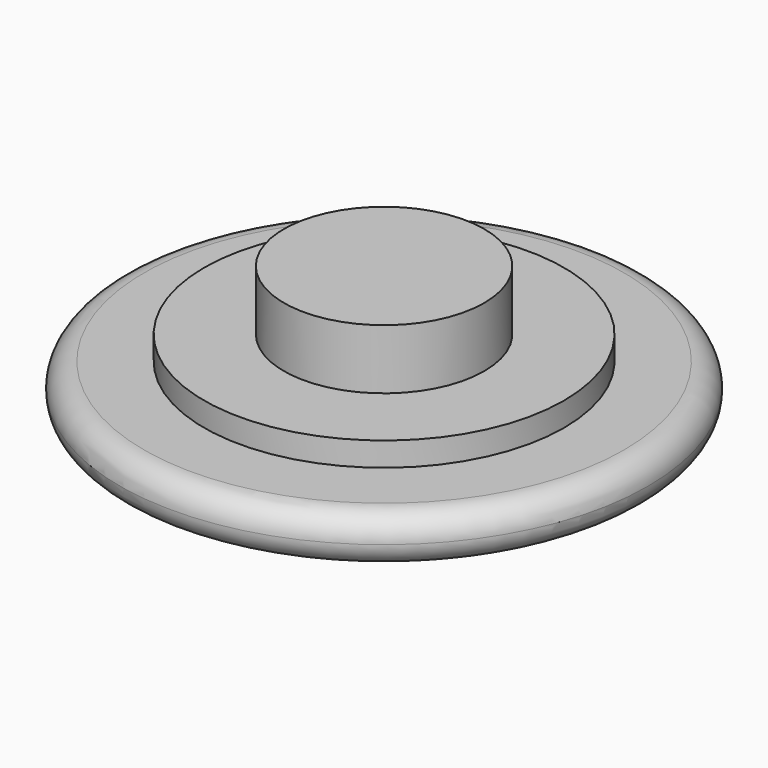
from build123d import *

# Parameters (mm, degrees)
F0_R         = 11
F0_R_2       = 7.5
F1_DEPTH     = 2
F0_R_3       = 4.175
F2_DEPTH     = 3
F3_DEPTH     = 5.5
F4_R         = 0.99999
F5_TEXT_SIZE = 6.3923610263
F6_DEPTH     = 1


# Not quite as in the source:
# - a fillet or chamfer is up to 0.001 mm smaller than in the source, because OpenCascade refuses the exact size
# - Text() gives the source's letters only with a copy of the font that has no kerning and outlines rounded to 1/6400 em; it was checked with that copy


with BuildPart() as f1:
    # F0 (on Top) → F1 (new body)
    with BuildSketch(Plane.XY):
        Circle(F0_R)
        Circle(F0_R_2, mode=Mode.SUBTRACT)
    extrude(amount=F1_DEPTH)

    # F0 (on Top) → F2 (join)
    with BuildSketch(Plane.XY):
        Circle(F0_R_2)
        Circle(F0_R_3, mode=Mode.SUBTRACT)
    extrude(amount=F2_DEPTH)

    # F0 (on Top) → F3 (join)
    with BuildSketch(Plane.XY):
        Circle(F0_R_3)
    extrude(amount=F3_DEPTH)

    # F4 (radius 1 in the source; OpenCascade refuses exactly that, so slightly less here)
    f4_edges = [f1.edges().sort_by_distance(p)[0] for p in [
        (-11, 0, 2),
        (-11, 0, 0),
    ]]
    fillet(f4_edges, radius=F4_R)

    # F5 (on face) → F6 (cut)
    with BuildSketch(Plane(origin=(0, 0, 0), x_dir=(1, 0, 0), z_dir=(0, 0, -1))):
        with Locations((-9.7998534976, -1.9906962162)):
            Text('Colton', F5_TEXT_SIZE, font='Open Sans', text_align=(TextAlign.LEFT, TextAlign.BOTTOM))
    extrude(amount=-F6_DEPTH, mode=Mode.SUBTRACT)


solid = f1.part
